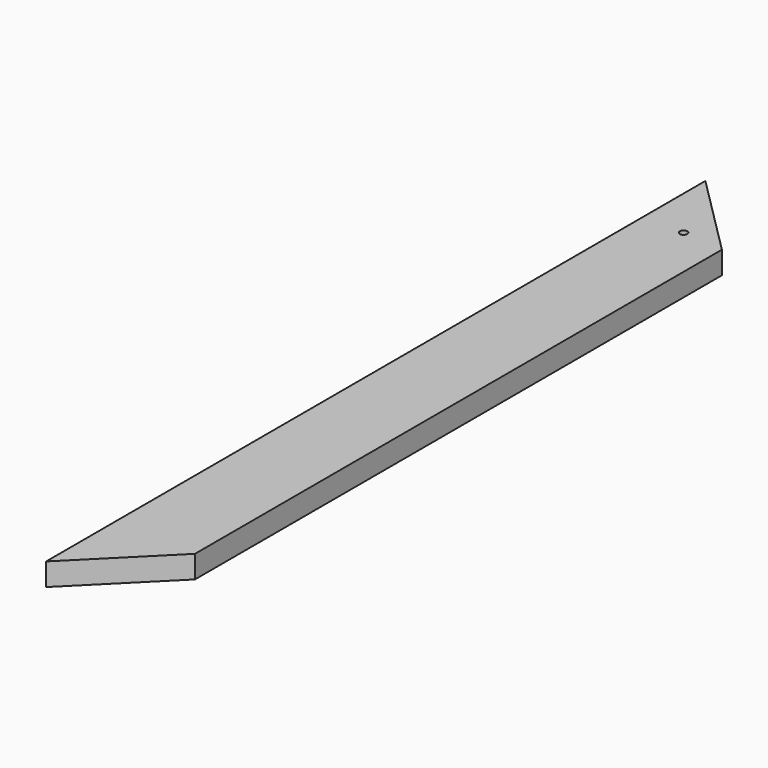
from build123d import *

# Parameters (mm, degrees)
F0_W      = 139.7
F0_H      = 38.1
F1_DEPTH  = 1828.8
F3_W      = 331.3202857971
F3_H      = 260.5838701129
F4_DEPTH  = 101.6
F7_W      = 1553.4552037716
F7_H      = 1155.3529500961
F8_DEPTH  = 762
F9_R      = 6.35
F10_DEPTH = 38.101


with BuildPart() as f1:
    # F0 (on Front) → F1 (new body)
    with BuildSketch(Plane.XZ):
        with Locations((69.85, 19.05)):
            Rectangle(F0_W, F0_H)
    extrude(amount=F1_DEPTH)

    # F3 (on face) → F4 (cut)
    with BuildSketch(Plane(origin=(984.25, -984.25, 0), x_dir=(-0.7071067812, -0.7071067812, 0), z_dir=(-0.7071067812, 0.7071067812, 0))):
        with Locations((1222.6701974869, 7.0506222546)):
            Rectangle(F3_W, F3_H)
    extrude(amount=F4_DEPTH, mode=Mode.SUBTRACT)

    # F7 (on face) → F8 (cut)
    with BuildSketch(Plane(origin=(-216.4381016486, -216.4381016486, 0), x_dir=(0.7071067812, -0.7071067812, 0), z_dir=(-0.7071067812, -0.7071067812, 0))):
        with Locations((614.4417077303, -181.5140247345)):
            Rectangle(F7_W, F7_H)
    extrude(amount=-F8_DEPTH, mode=Mode.SUBTRACT)

    # F9 (on face) → F10 (cut, through all)
    with BuildSketch(Plane.XY.offset(38.1)):
        with Locations((69.85, -566.2262032972)):
            Circle(F9_R)
    extrude(amount=-F10_DEPTH, mode=Mode.SUBTRACT)


solid = f1.part
